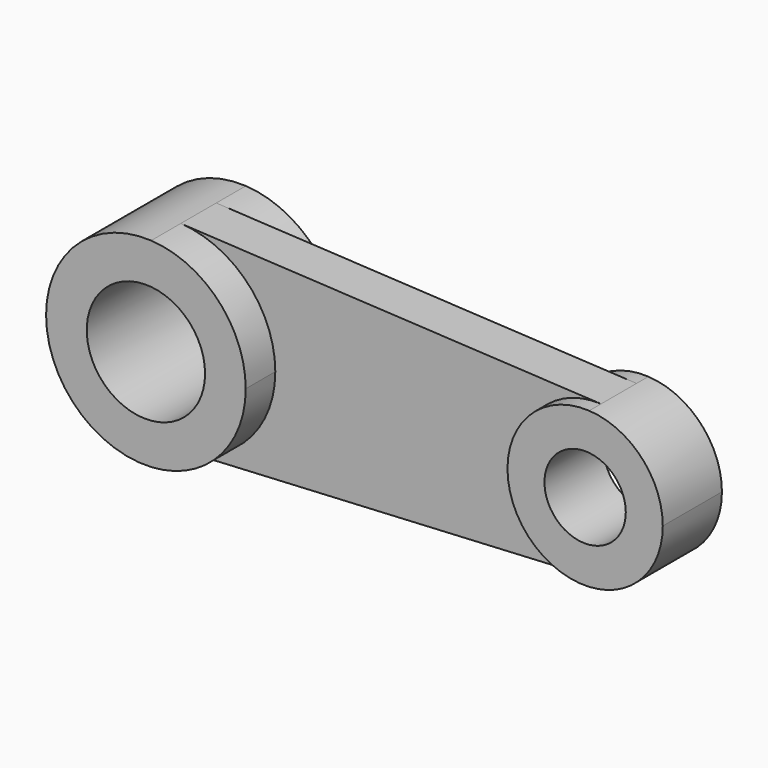
from build123d import *

# Parameters (mm, degrees)
F0_R     = 25.4
F1_DEPTH = 25.4
F0_R_2   = 17.4625
F2_DEPTH = 15.875
F3_DEPTH = 9.525


with BuildPart() as f1:
    # F0 (on Front) → F1 (new body, symmetric)
    with BuildSketch(Plane.XZ):
        with BuildLine():
            ThreePointArc((2.255921, -42.803092), (31.095726, -29.499996), (42.8625, 0))
            ThreePointArc((42.8625, 0), (31.095726, 29.499996), (2.255921, 42.803092))
            ThreePointArc((2.255921, 42.803092), (-42.8625, 0), (2.255921, -42.803092))
        make_face()
        Circle(F0_R, mode=Mode.SUBTRACT)
    extrude(amount=F1_DEPTH, both=True)



with BuildPart() as f2:
    # F0 (on Front) → F2 (new body, symmetric)
    with BuildSketch(Plane.XZ):
        with BuildLine():
            ThreePointArc((214.3125, 0), (205.160564, 22.944441), (182.729605, 33.291294))
            ThreePointArc((182.729605, 33.291294), (147.6375, 0), (182.729605, -33.291294))
            ThreePointArc((182.729605, -33.291294), (205.160564, -22.944441), (214.3125, 0))
        make_face()
        with Locations((180.975, 0)):
            Circle(F0_R_2, mode=Mode.SUBTRACT)
    extrude(amount=F2_DEPTH, both=True)


with BuildPart() as f1_1:
    add(f1.part)

    add(f2.part)  # F3 merges F2
    # F0 (on Front) → F3 (join, symmetric)
    with BuildSketch(Plane.XZ):
        with BuildLine():
            ThreePointArc((2.255921, 42.803092), (31.095726, 29.499996), (42.8625, 0))
            ThreePointArc((42.8625, 0), (31.095726, -29.499996), (2.255921, -42.803092))
            Line((2.255921, -42.803092), (182.729605, -33.291294))
            ThreePointArc((182.729605, -33.291294), (147.6375, 0), (182.729605, 33.291294))
            Line((182.729605, 33.291294), (2.255921, 42.803092))
        make_face()
    extrude(amount=F3_DEPTH, both=True)


solid = f1_1.part
